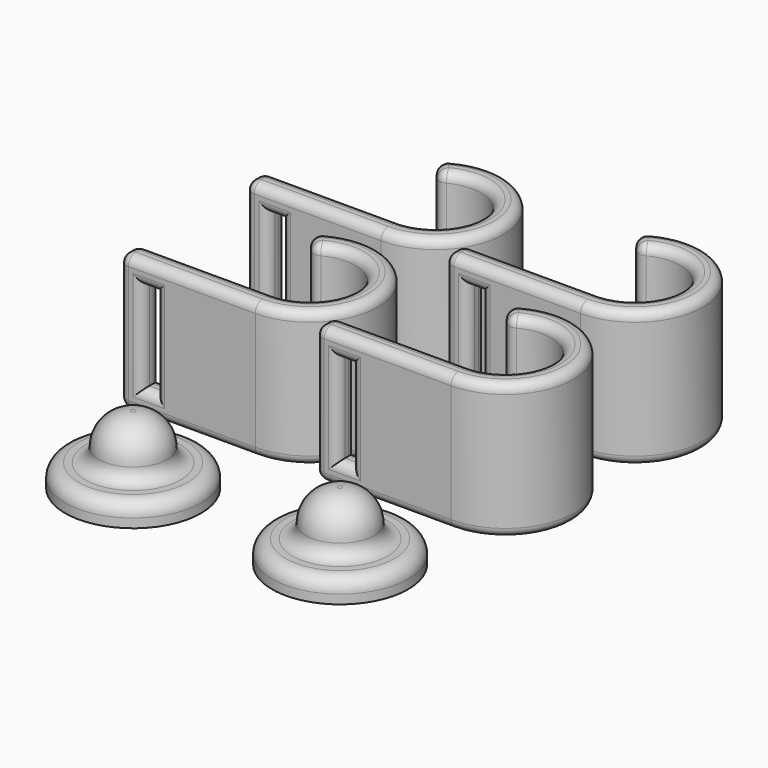
from build123d import *

# Parameters (mm, degrees)
F1_DEPTH  = 30
F2_W      = 3
F2_H      = 20
F3_DEPTH  = 25
F4_R      = 2
F8_R      = 7.5
F9_DEPTH  = 15
F10_R     = 7
F8_R_2    = 15
F11_DEPTH = 5
F12_R     = 2.99999


# Not quite as in the source:
# - a fillet or chamfer is up to 0.001 mm smaller than in the source, because OpenCascade refuses the exact size


with BuildPart() as f1:
    # F0 (on Top) → F1 (new body)
    with BuildSketch(Plane.XY):
        with BuildLine():
            ThreePointArc((-5.8989744072, 8.0747817892), (9.5065192866, 3.1025942458), (0, -10))
            Line((0, -10), (-30, -10))
            Line((-30, -10), (-30, -15))
            Line((-30, -15), (0, -15))
            ThreePointArc((0, -15), (14.1565356299, 4.9590824714), (-9.3604570265, 11.7210001389))
            Line((-9.3604570265, 11.7210001389), (-5.8989744072, 8.0747817892))
        make_face()
    extrude(amount=F1_DEPTH)

    # F2 (on face) → F3 (cut)
    with BuildSketch(Plane.XZ.offset(15)):
        with Locations((-23.5, 15)):
            Rectangle(F2_W, F2_H)
    extrude(amount=-F3_DEPTH, mode=Mode.SUBTRACT)

    # F4
    f4_edges = [f1.edges().sort_by_distance(p)[0] for p in [
        (9.506519, 3.102594, 30),
        (-15, -10, 30),
        (-30, -12.5, 30),
        (-15, -15, 30),
        (14.156536, 4.959082, 30),
        (-7.629716, 9.897891, 30),
        (9.506519, 3.102594, 0),
        (-15, -10, 0),
        (-30, -12.5, 0),
        (-15, -15, 0),
        (14.156536, 4.959082, 0),
        (-7.629716, 9.897891, 0),
        (-30, -10, 15),
        (-30, -15, 15),
        (-9.360457, 11.721, 15),
        (-5.898974, 8.074782, 15),
        (-22, -15, 15),
        (-25, -15, 15),
        (-23.5, -15, 5),
        (-23.5, -15, 25),
        (0, -10, 15),
        (-23.5, -10, 25),
        (-25, -10, 15),
        (-23.5, -10, 5),
        (-22, -10, 15),
    ]]
    fillet(f4_edges, radius=F4_R)


with BuildPart() as f5_1:
    # F5: copy of F1
    add(f1.part.moved(Location((0, 34.7, 0))))


with BuildPart() as f6_1:
    # F6: copy of F1
    add(f1.part.moved(Location((43.2, 0, 0))))


with BuildPart() as f7_1:
    # F7: copy of F6_1
    add(f6_1.part.moved(Location((0.6, 35, 0))))


with BuildPart() as f9:
    # F8 (on Top) → F9 (new body)
    with BuildSketch(Plane.XY):
        with Locations((36.2773165107, -36.9656942785)):
            Circle(F8_R)
    extrude(amount=F9_DEPTH)

    # F10
    f10_edges = [f9.edges().sort_by_distance(p)[0] for p in [
        (28.777317, -36.965694, 15),
    ]]
    fillet(f10_edges, radius=F10_R)

    # F8 (on Top) → F11 (join)
    with BuildSketch(Plane.XY):
        with Locations((36.2773165107, -36.9656942785)):
            Circle(F8_R_2)
        with Locations((36.2773165107, -36.9656942785)):
            Circle(F8_R, mode=Mode.SUBTRACT)
    extrude(amount=F11_DEPTH)

    # F12 (radius 3 in the source; OpenCascade refuses exactly that, so slightly less here)
    f12_edges = [f9.edges().sort_by_distance(p)[0] for p in [
        (21.277317, -36.965694, 5),
        (28.777317, -36.965694, 5),
    ]]
    fillet(f12_edges, radius=F12_R)


with BuildPart() as f13_1:
    # F13: copy of F9
    add(f9.part.moved(Location((-45.6, -0.1, 0))))


solid = Compound([f1.part, f5_1.part, f6_1.part, f7_1.part, f9.part, f13_1.part])
